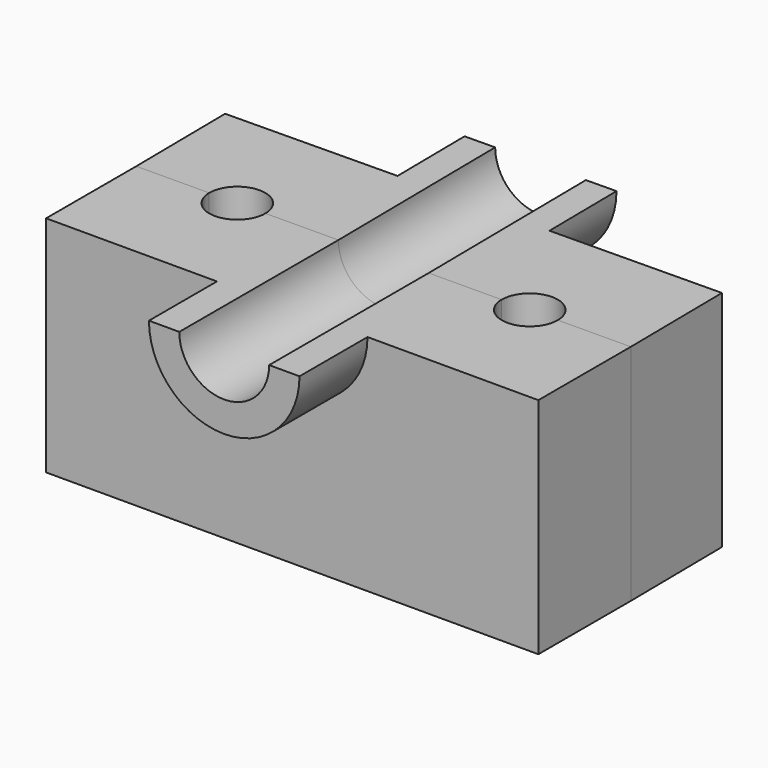
from build123d import *
from build123d import SkipClean  # not in build123d's __all__

# Parameters (mm, degrees)
F1_DEPTH = 50.8
F3_DEPTH = 33.782
F4_DEPTH = 19.304
F7_DEPTH = 62.738
F8_DEPTH = 50.8


with BuildPart() as f1:
    # F0 (on Top) → F1 (new body)
    with BuildSketch(Plane.XY):
        Polygon((-50.1712188125, 0), (-50.1712188125, -25.5924221128), (61.6167448461, -25.5924221128), (61.6167448461, 0.6504831836), align=None)
    extrude(amount=F1_DEPTH)

    # F2 (on face) → F3 (cut)
    with BuildSketch(Plane.XZ.offset(25.5924221128)):
        with BuildLine():
            Line((15.9283644421, 50.8), (-4.4828384085, 50.8))
            ThreePointArc((-4.4828384085, 50.8), (5.7227630168, 40.5943985747), (15.9283644421, 50.8))
        make_face()
    extrude(amount=-F3_DEPTH, mode=Mode.SUBTRACT)

    # F2 (on face) → F4 (join)
    with BuildSketch(Plane.XZ.offset(25.5924221128)):
        with BuildLine():
            Line((-4.4828384085, 50.8), (-11.371643244, 50.8))
            ThreePointArc((-11.371643244, 50.8), (5.7227630168, 33.7055937392), (22.8171692776, 50.8))
            Line((22.8171692776, 50.8), (15.9283644421, 50.8))
            ThreePointArc((15.9283644421, 50.8), (5.7227630168, 40.5943985747), (-4.4828384085, 50.8))
        make_face()
    extrude(amount=F4_DEPTH)

    # F5 (on face) → F7 (cut)
    with BuildSketch(Plane.XY.offset(50.8)):
        with BuildLine():
            Line((-20.977136112, 0.1698775005), (-33.6769211089, 0.0959786987))
            ThreePointArc((-33.6769211089, 0.0959786987), (-27.2900792096, -6.2169643988), (-20.977136112, 0.1698775005))
        make_face()
    extrude(amount=-F7_DEPTH, mode=Mode.SUBTRACT)

    # F6 (on face) → F8 (cut)
    with BuildSketch(Plane.XY.offset(50.8)):
        with BuildLine():
            Line((45.1224471426, 0.5545044849), (32.4226621457, 0.480605683))
            ThreePointArc((32.4226621457, 0.480605683), (38.809504045, -5.8323374145), (45.1224471426, 0.5545044849))
        make_face()
    extrude(amount=-F8_DEPTH, mode=Mode.SUBTRACT)

    # F9: F1 across face


with BuildPart() as f1_1:
    add(f1.part, clean=False)
    with SkipClean():  # cleaning this boolean's faces spoils the solid; the shape is the same uncleaned
        add(f1.part.mirror(Plane(origin=(5.7227630168, 0.3252415918, 24.0477864572), x_dir=(-0.9999830706, -0.0058188033, 0), z_dir=(-0.0058188033, 0.9999830706, 0))), clean=False)


solid = f1_1.part
